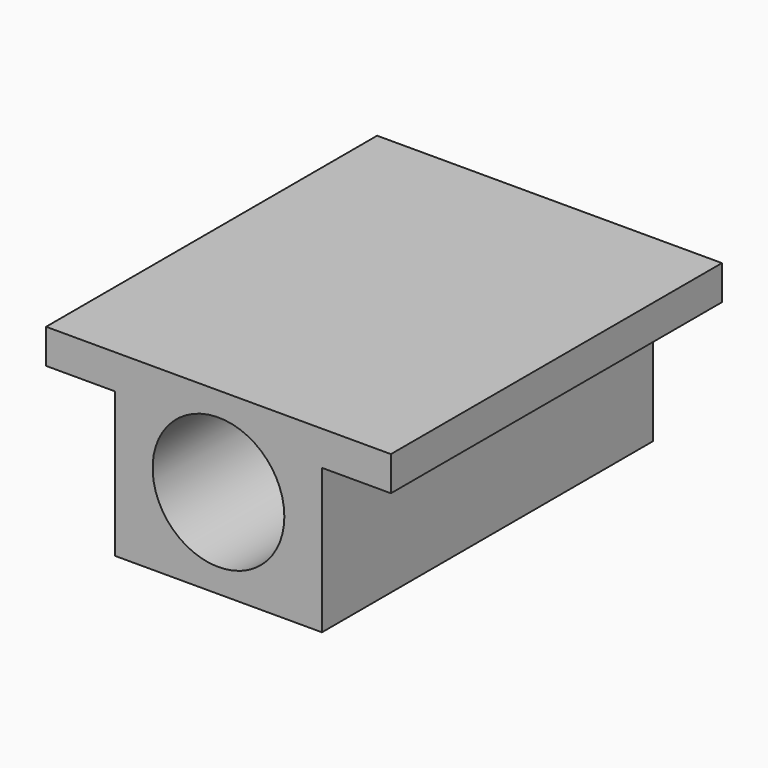
from build123d import *

# Parameters (mm, degrees)
F0_W     = 63.5
F0_H     = 76.2
F1_DEPTH = 33.02
F2_R     = 12.1285
F3_DEPTH = 100.076
F4_W     = 12.7
F4_H     = 26.67
F5_DEPTH = 76.201


# Not quite as in the source:
# - a feature names something its author has since deleted; it is built from what else it names


with BuildPart() as f1:
    # F0 (on Top) → F1 (new body)
    with BuildSketch(Plane.XY):
        Rectangle(F0_W, F0_H)
    extrude(amount=F1_DEPTH)

    # F2 (on face) → F3 (cut)
    with BuildSketch(Plane.XZ.offset(38.1)):
        with Locations((0, 16.51)):
            Circle(F2_R)
    extrude(amount=-F3_DEPTH, mode=Mode.SUBTRACT)

    # F4 (on face) → F5 (cut, through all)
    with BuildSketch(Plane.XZ.offset(38.1)):
        with Locations((25.4, 13.335)):
            Rectangle(F4_W, F4_H)
        with Locations((-25.4, 13.335)):
            Rectangle(F4_W, F4_H)
    extrude(amount=-F5_DEPTH, mode=Mode.SUBTRACT)


solid = f1.part
